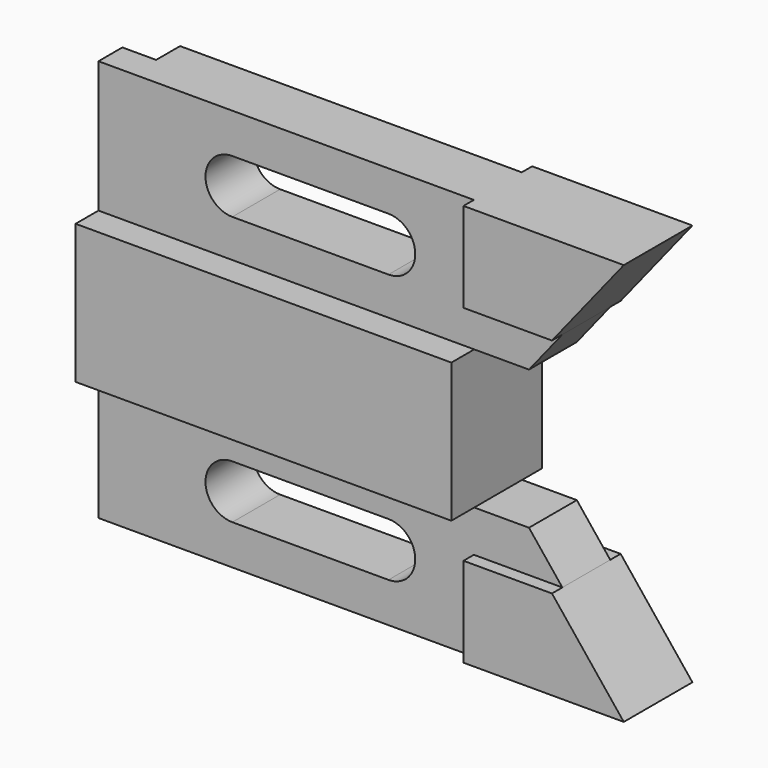
from build123d import *

# Parameters (mm, degrees)
F1_DEPTH = 22.098
F4_DEPTH = 5.842
F5_DEPTH = 8.382
F3_W     = 6.592599522
F3_H     = 25.6785105251
F6_DEPTH = 5.842
F7_DEPTH = 5.842


with BuildPart() as f1:
    # F0 (on Front) → F1 (new body)
    with BuildSketch(Plane.XZ):
        Polygon((-38.0060652603, 0), (35.3999347397, 0), (35.3999347397, 27.1923393011), (-38.0060652603, 27.1923393011), (-38.0060652603, 18.1223209947), (-38.0060652603, 10.0105842575), align=None)
    extrude(amount=F1_DEPTH)

    # F3 (on offset) → F4 (join, symmetric)
    with BuildSketch(Plane.XZ.offset(10.668)):
        Polygon((35.3301167488, 0), (-31.4134657383, 0), (-31.4134657383, -25.6785105251), (35.3301167488, -25.6785105251), (35.3301167488, -8.1525105251), (52.6165383837, -8.1525105251), (46.0923918922, 0), align=None)
        with BuildLine():
            Line((18.6442192644, -17.8938459214), (-11.8596823886, -17.8938459214))
            ThreePointArc((-11.8596823886, -17.8938459214), (-17.0929335328, -12.6605947772), (-11.8596823886, -7.427343633))
            Line((-11.8596823886, -7.427343633), (18.6442192644, -7.427343633))
            ThreePointArc((18.6442192644, -7.427343633), (23.8774704086, -12.6605947772), (18.6442192644, -17.8938459214))
        make_face(mode=Mode.SUBTRACT)
        Polygon((-31.4134657383, 52.8708498262), (-31.4134657383, 27.1923393011), (46.0923918922, 27.1923393011), (52.6165383837, 35.3448498262), (35.3301167488, 35.3448498262), (35.3301167488, 52.8708498262), align=None)
        with BuildLine():
            ThreePointArc((18.6442192644, 45.0756415895), (23.8774704086, 39.8423904453), (18.6442192644, 34.6091393011))
            Line((18.6442192644, 34.6091393011), (-11.8596823886, 34.6091393011))
            ThreePointArc((-11.8596823886, 34.6091393011), (-17.0929335328, 39.8423904453), (-11.8596823886, 45.0756415895))
            Line((-11.8596823886, 45.0756415895), (18.6442192644, 45.0756415895))
        make_face(mode=Mode.SUBTRACT)
    extrude(amount=F4_DEPTH, both=True)

    # F3 (on offset) → F5 (join, symmetric)
    with BuildSketch(Plane.XZ.offset(10.668)):
        Polygon((35.3301167488, -8.1525105251), (35.3301167488, -25.6785105251), (66.6419347397, -25.6785105251), (52.6165383837, -8.1525105251), align=None)
        Polygon((35.3301167488, 35.3448498262), (52.6165383837, 35.3448498262), (66.6419347397, 52.8708498262), (35.3301167488, 52.8708498262), align=None)
    extrude(amount=F5_DEPTH, both=True)

    # F3 (on offset) → F6 (join, through all)
    with BuildSketch(Plane.XZ.offset(10.668)):
        with Locations((-34.7097654993, -12.8392552625)):
            Rectangle(F3_W, F3_H)
    extrude(amount=F6_DEPTH)

    # F3 (on offset) → F7 (join, through all)
    with BuildSketch(Plane.XZ.offset(10.668)):
        with Locations((-34.7097654993, 40.0315945636)):
            Rectangle(F3_W, F3_H)
    extrude(amount=F7_DEPTH)


solid = f1.part
